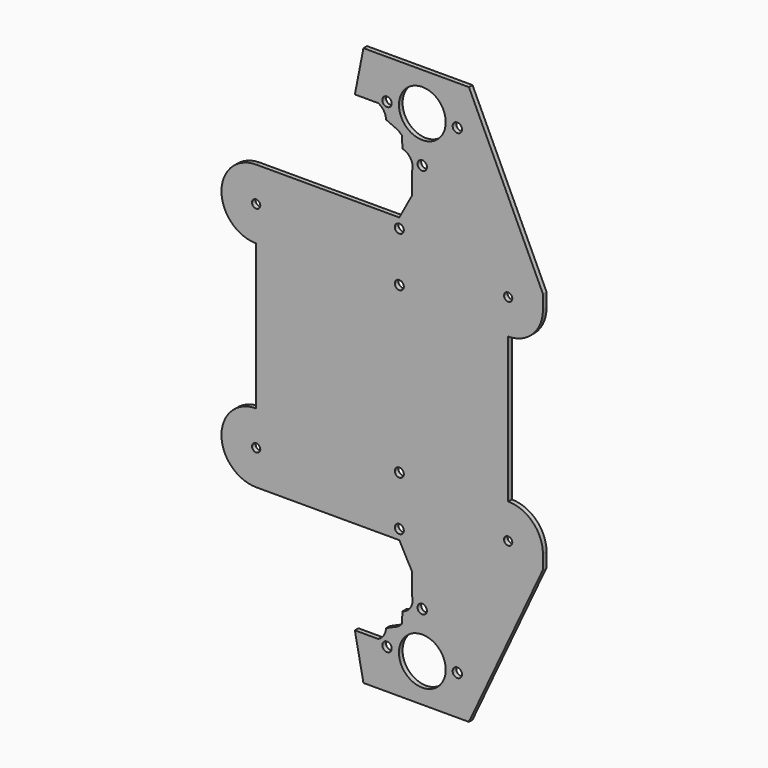
from build123d import *

# Parameters (mm, degrees)
F0_R     = 3.302
F0_R_2   = 16.51
F0_W     = 177.8
F0_H     = 77.7875
F1_DEPTH = 3.175


# Not quite as in the source:
# - ends of sketch curves that miss each other by under 0.0002 mm in the source are joined


with BuildPart() as f1:
    # F0 (on Front) → F1 (new body)
    with BuildSketch(Plane.XZ):
        with BuildLine():
            Line((-4.6405893252, -64.494198626), (72.172606051, -64.494198626))
            ThreePointArc((72.172606051, -64.494198626), (89.5045003647, -57.3150929397), (96.683606051, -39.983198626))
            Line((96.683606051, -39.983198626), (96.683606051, -30.0584486086))
            Line((96.683606051, -30.0584486086), (44.4719158113, 81.3992435336))
            Line((44.4719158113, 81.3992435336), (-29.9480052508, 81.3992435336))
            Line((-29.9480052508, 81.3992435336), (-35.9978974571, 50.6829957967))
            Line((-35.9978974571, 50.6829957967), (-19.4879078689, 50.6714224456))
            ThreePointArc((-19.4879078689, 50.6714224456), (-15.5812211009, 47.1637298884), (-13.9720730804, 42.1660573792))
            Line((-13.9720730804, 42.1660573792), (-5.4024819992, 38.3506346508))
            Line((-5.4024819992, 38.3506346508), (-2.9009456417, 36.1038269705))
            Line((-2.9009456417, 36.1038269705), (-2.3647786124, 27.9011076368))
            ThreePointArc((-2.3647786124, 27.9011076368), (3.4353485173, 23.5426794776), (4.3712937617, 16.3481414632))
            Line((4.3712937617, 16.3481414632), (4.2880776677, 1.0115236557))
            Line((4.2880776677, 1.0115236557), (-4.6405893252, -15.5276898319))
            Line((-4.6405893252, -15.5276898319), (-105.627393949, -15.5276898319))
            ThreePointArc((-105.627393949, -15.5276898319), (-130.1106483461, -40.010944229), (-105.627393949, -64.494198626))
            Line((-105.627393949, -64.494198626), (-4.6405893252, -64.494198626))
        make_face()
        with BuildLine():
            ThreePointArc((-105.627393949, -37.1117488528), (-103.5773532385, -37.9609035185), (-102.7281985728, -40.010944229))
            ThreePointArc((-102.7281985728, -40.010944229), (-103.5773532385, -42.0609849395), (-105.627393949, -42.9101396052))
            ThreePointArc((-105.627393949, -42.9101396052), (-107.6774346595, -42.0609849395), (-108.5265893252, -40.010944229))
            ThreePointArc((-108.5265893252, -40.010944229), (-107.6774346595, -37.9609035185), (-105.627393949, -37.1117488528))
        make_face(mode=Mode.SUBTRACT)
        with BuildLine():
            ThreePointArc((-4.6405893252, -54.334198626), (-2.3955252949, -55.2641345958), (-1.4655893252, -57.509198626))
            ThreePointArc((-1.4655893252, -57.509198626), (-2.3955252949, -59.7542626563), (-4.6405893252, -60.684198626))
            ThreePointArc((-4.6405893252, -60.684198626), (-6.8856533555, -59.7542626563), (-7.8155893252, -57.509198626))
            ThreePointArc((-7.8155893252, -57.509198626), (-6.8856533555, -55.2641345958), (-4.6405893252, -54.334198626))
        make_face(mode=Mode.SUBTRACT)
        with BuildLine():
            ThreePointArc((-4.6405893252, -19.282198626), (-2.3955252949, -20.2121345958), (-1.4655893252, -22.457198626))
            ThreePointArc((-1.4655893252, -22.457198626), (-2.3955252949, -24.7022626563), (-4.6405893252, -25.632198626))
            ThreePointArc((-4.6405893252, -25.632198626), (-6.8856533555, -24.7022626563), (-7.8155893252, -22.457198626))
            ThreePointArc((-7.8155893252, -22.457198626), (-6.8856533555, -20.2121345958), (-4.6405893252, -19.282198626))
        make_face(mode=Mode.SUBTRACT)
        with BuildLine():
            ThreePointArc((72.172606051, -37.0840032499), (74.2226467615, -37.9331579156), (75.0718014272, -39.983198626))
            ThreePointArc((75.0718014272, -39.983198626), (74.2226467615, -42.0332393365), (72.172606051, -42.8823940022))
            ThreePointArc((72.172606051, -42.8823940022), (70.1225653405, -42.0332393365), (69.2734106748, -39.983198626))
            ThreePointArc((69.2734106748, -39.983198626), (70.1225653405, -37.9331579156), (72.172606051, -37.0840032499))
        make_face(mode=Mode.SUBTRACT)
        with Locations((11.5432352797, 22.0017248669)):
            Circle(F0_R, mode=Mode.SUBTRACT)
        with Locations((-13.3156779021, 53.5307241817)):
            Circle(F0_R, mode=Mode.SUBTRACT)
        with Locations((11.6086210255, 54.3104703533)):
            Circle(F0_R_2, mode=Mode.SUBTRACT)
        with Locations((36.2912922688, 53.4994019413)):
            Circle(F0_R, mode=Mode.SUBTRACT)
        Polygon((72.172606051, -76.841138626), (72.172606051, -64.494198626), (-4.6405893252, -64.494198626), (-105.627393949, -64.494198626), (-105.627393949, -76.841138626), align=None)
        with Locations((-16.727393949, -115.734888626)):
            Rectangle(F0_W, F0_H)
        Polygon((72.172606051, -166.975578626), (72.172606051, -154.628638626), (-105.627393949, -154.628638626), (-105.627393949, -166.975578626), (-4.6405893252, -166.975578626), align=None)
        with BuildLine():
            ThreePointArc((96.683606051, -191.486578626), (89.5045003647, -174.1546843124), (72.172606051, -166.975578626))
            Line((72.172606051, -166.975578626), (-4.6405893252, -166.975578626))
            Line((-4.6405893252, -166.975578626), (-105.627393949, -166.975578626))
            ThreePointArc((-105.627393949, -166.975578626), (-130.1106483461, -191.4588330231), (-105.627393949, -215.9420874201))
            Line((-105.627393949, -215.9420874201), (-4.6405893252, -215.9420874201))
            Line((-4.6405893252, -215.9420874201), (4.2880776677, -232.4813009078))
            Line((4.2880776677, -232.4813009078), (4.3712937617, -247.8179187153))
            ThreePointArc((4.3712937617, -247.8179187153), (3.4353485173, -255.0124567297), (-2.3647786124, -259.3708848889))
            Line((-2.3647786124, -259.3708848889), (-2.9009456417, -267.5736042226))
            Line((-2.9009456417, -267.5736042226), (-5.4024819992, -269.8204119029))
            Line((-5.4024819992, -269.8204119029), (-13.9720735102, -273.635839865))
            ThreePointArc((-13.9720735102, -273.635839865), (-15.5812211009, -278.6335071405), (-19.487905219, -282.1411996959))
            Line((-19.487905219, -282.1411996959), (-35.9978974571, -282.1527730488))
            Line((-35.9978974571, -282.1527730488), (-29.9480052508, -312.8690207857))
            Line((-29.9480052508, -312.8690207857), (44.4719158113, -312.8690207857))
            Line((44.4719158113, -312.8690207857), (96.683606051, -201.4113286435))
            Line((96.683606051, -201.4113286435), (96.683606051, -191.486578626))
        make_face()
        with BuildLine():
            ThreePointArc((-105.627393949, -194.3580283993), (-107.6774346595, -193.5088737336), (-108.5265893252, -191.4588330231))
            ThreePointArc((-108.5265893252, -191.4588330231), (-107.6774346595, -189.4087923126), (-105.627393949, -188.5596376469))
            ThreePointArc((-105.627393949, -188.5596376469), (-103.5773532385, -189.4087923126), (-102.7281985728, -191.4588330231))
            ThreePointArc((-102.7281985728, -191.4588330231), (-103.5773532385, -193.5088737336), (-105.627393949, -194.3580283993))
        make_face(mode=Mode.SUBTRACT)
        with Locations((-13.3156779021, -285.0005014338)):
            Circle(F0_R, mode=Mode.SUBTRACT)
        with Locations((11.6086210255, -285.7802476054)):
            Circle(F0_R_2, mode=Mode.SUBTRACT)
        with Locations((36.2912922688, -284.9691791934)):
            Circle(F0_R, mode=Mode.SUBTRACT)
        with Locations((11.5432352796, -253.471502119)):
            Circle(F0_R, mode=Mode.SUBTRACT)
        with BuildLine():
            ThreePointArc((-1.4655893252, -209.012578626), (-2.3955252949, -211.2576426563), (-4.6405893252, -212.187578626))
            ThreePointArc((-4.6405893252, -212.187578626), (-6.8856533555, -211.2576426563), (-7.8155893252, -209.012578626))
            ThreePointArc((-7.8155893252, -209.012578626), (-6.8856533555, -206.7675145958), (-4.6405893252, -205.837578626))
            ThreePointArc((-4.6405893252, -205.837578626), (-2.3955252949, -206.7675145958), (-1.4655893252, -209.012578626))
        make_face(mode=Mode.SUBTRACT)
        with BuildLine():
            ThreePointArc((-1.4655893252, -173.960578626), (-2.3955252949, -176.2056426563), (-4.6405893252, -177.135578626))
            ThreePointArc((-4.6405893252, -177.135578626), (-6.8856533555, -176.2056426563), (-7.8155893252, -173.960578626))
            ThreePointArc((-7.8155893252, -173.960578626), (-6.8856533555, -171.7155145958), (-4.6405893252, -170.785578626))
            ThreePointArc((-4.6405893252, -170.785578626), (-2.3955252949, -171.7155145958), (-1.4655893252, -173.960578626))
        make_face(mode=Mode.SUBTRACT)
        with BuildLine():
            ThreePointArc((72.172606051, -194.3857740022), (70.1225653405, -193.5366193365), (69.2734106748, -191.486578626))
            ThreePointArc((69.2734106748, -191.486578626), (70.1225653405, -189.4365379156), (72.172606051, -188.5873832499))
            ThreePointArc((72.172606051, -188.5873832499), (74.2226467615, -189.4365379156), (75.0718014272, -191.486578626))
            ThreePointArc((75.0718014272, -191.486578626), (74.2226467615, -193.5366193365), (72.172606051, -194.3857740022))
        make_face(mode=Mode.SUBTRACT)
    extrude(amount=F1_DEPTH)


solid = f1.part
